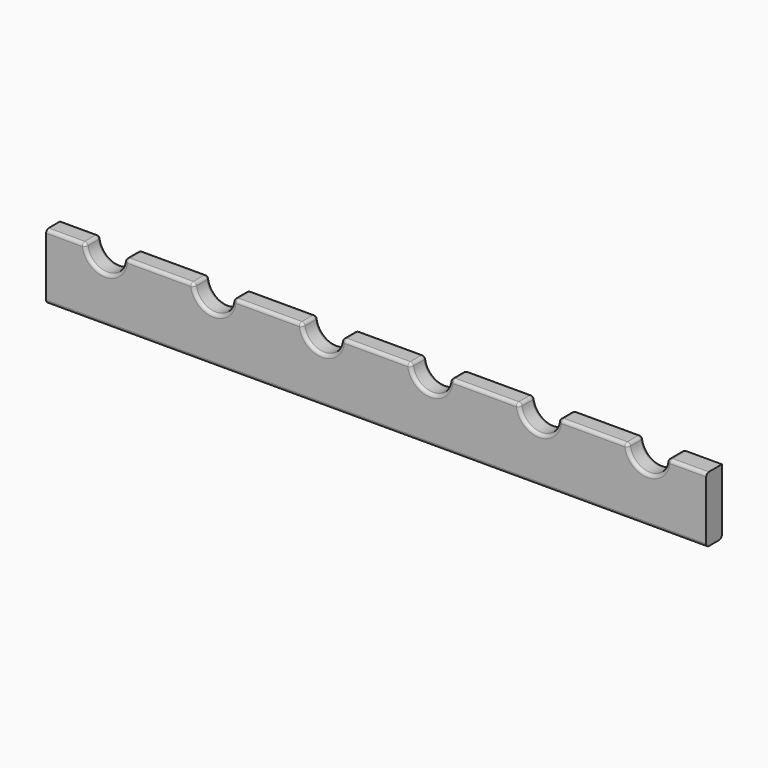
from build123d import *

# Parameters (mm, degrees)
F1_DEPTH = 19.05
F2_R     = 3.175
F3_R     = 3.175


with BuildPart() as f1:
    # F0 (on Front) → F1 (new body)
    with BuildSketch(Plane.XZ):
        with BuildLine():
            Line((-320.675, 31.75), (-320.675, -31.75))
            Line((-320.675, -31.75), (320.675, -31.75))
            Line((320.675, -31.75), (320.675, 31.75))
            Line((320.675, 31.75), (282.575, 31.75))
            ThreePointArc((282.575, 31.75), (263.525, 12.7), (244.475, 31.75))
            Line((244.475, 31.75), (177.165, 31.75))
            ThreePointArc((177.165, 31.75), (158.115, 12.7), (139.065, 31.75))
            Line((139.065, 31.75), (71.755, 31.75))
            ThreePointArc((71.755, 31.75), (52.705, 12.7), (33.655, 31.75))
            Line((33.655, 31.75), (-33.655, 31.75))
            ThreePointArc((-33.655, 31.75), (-52.705, 12.7), (-71.755, 31.75))
            Line((-71.755, 31.75), (-139.065, 31.75))
            ThreePointArc((-139.065, 31.75), (-158.115, 12.7), (-177.165, 31.75))
            Line((-177.165, 31.75), (-244.475, 31.75))
            ThreePointArc((-244.475, 31.75), (-263.525, 12.7), (-282.575, 31.75))
            Line((-282.575, 31.75), (-320.675, 31.75))
        make_face()
    extrude(amount=-F1_DEPTH)

    # F2
    f2_edges = [f1.edges().sort_by_distance(p)[0] for p in [
        (-244.475, 9.525, 31.75),
        (-282.575, 9.525, 31.75),
        (-263.525, 0, 12.7),
        (-263.525, 19.05, 12.7),
        (-301.625, 0, 31.75),
        (-301.625, 19.05, 31.75),
        (-177.165, 9.525, 31.75),
        (-210.82, 0, 31.75),
        (-210.82, 19.05, 31.75),
        (-139.065, 9.525, 31.75),
        (-158.115, 0, 12.7),
        (-158.115, 19.05, 12.7),
        (-71.755, 9.525, 31.75),
        (-105.41, 0, 31.75),
        (-105.41, 19.05, 31.75),
        (-33.655, 9.525, 31.75),
        (-52.705, 0, 12.7),
        (-52.705, 19.05, 12.7),
        (33.655, 9.525, 31.75),
        (0, 0, 31.75),
        (0, 19.05, 31.75),
        (71.755, 9.525, 31.75),
        (52.705, 0, 12.7),
        (52.705, 19.05, 12.7),
        (139.065, 9.525, 31.75),
        (105.41, 0, 31.75),
        (105.41, 19.05, 31.75),
        (177.165, 9.525, 31.75),
        (158.115, 0, 12.7),
        (158.115, 19.05, 12.7),
        (244.475, 9.525, 31.75),
        (210.82, 0, 31.75),
        (210.82, 19.05, 31.75),
        (282.575, 9.525, 31.75),
        (263.525, 0, 12.7),
        (263.525, 19.05, 12.7),
        (301.625, 0, 31.75),
    ]]
    fillet(f2_edges, radius=F2_R)

    # F3
    f3_edges = [f1.edges().sort_by_distance(p)[0] for p in [
        (0, 0, -31.75),
        (0, 19.05, -31.75),
    ]]
    fillet(f3_edges, radius=F3_R)


solid = f1.part
